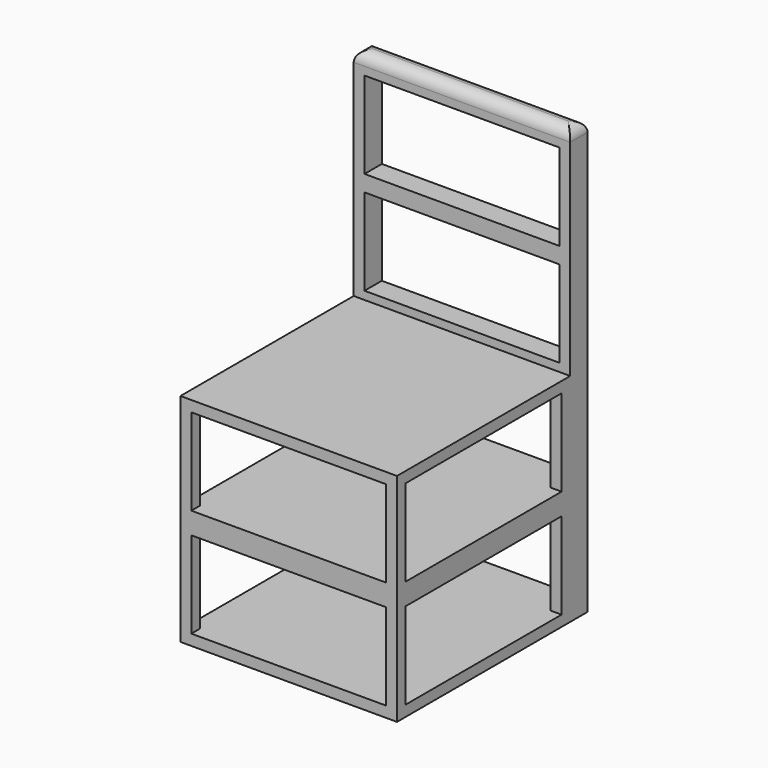
from build123d import *

# Parameters (mm, degrees)
F0_W     = 50
F0_H     = 5
F1_DEPTH = 100
F0_H_2   = 50
F2_DEPTH = 50
F3_W     = 22.5
F3_H     = 20
F4_DEPTH = 100
F5_W     = 22.5
F5_H     = 20
F6_DEPTH = 55
F7_R     = 2.49999
F8_W     = 45
F8_H     = 20
F9_DEPTH = 25


# Not quite as in the source:
# - a fillet or chamfer is up to 0.001 mm smaller than in the source, because OpenCascade refuses the exact size


with BuildPart() as f1:
    # F0 (on Top) → F1 (new body)
    with BuildSketch(Plane.XY):
        with Locations((0, 27.5)):
            Rectangle(F0_W, F0_H)
    extrude(amount=F1_DEPTH)

    # F0 (on Top) → F2 (join)
    with BuildSketch(Plane.XY):
        Rectangle(F0_W, F0_H_2)
    extrude(amount=F2_DEPTH)

    # F3 (on face) → F4 (cut)
    with BuildSketch(Plane.XZ.offset(25)):
        with Locations((-11.25, 37.5)):
            Rectangle(F3_W, F3_H)
        with Locations((11.25, 37.5)):
            Rectangle(F3_W, F3_H)
        with Locations((-11.25, 12.5)):
            Rectangle(F3_W, F3_H)
        with Locations((11.25, 12.5)):
            Rectangle(F3_W, F3_H)
    extrude(amount=-F4_DEPTH, mode=Mode.SUBTRACT)

    # F5 (on face) → F6 (cut)
    with BuildSketch(Plane(origin=(-25, 0, 0), x_dir=(0, -1, 0), z_dir=(-1, 0, 0))):
        with Locations((-11.25, 37.5)):
            Rectangle(F5_W, F5_H)
        with Locations((11.25, 37.5)):
            Rectangle(F5_W, F5_H)
        with Locations((11.25, 12.5)):
            Rectangle(F5_W, F5_H)
        with Locations((-11.25, 12.5)):
            Rectangle(F5_W, F5_H)
    extrude(amount=-F6_DEPTH, mode=Mode.SUBTRACT)

    # F7 (radius 2.5 in the source; OpenCascade refuses exactly that, so slightly less here)
    f7_edges = [f1.edges().sort_by_distance(p)[0] for p in [
        (0, 25, 100),
        (25, 27.5, 100),
        (0, 30, 100),
        (-25, 27.5, 100),
    ]]
    fillet(f7_edges, radius=F7_R)

    # F8 (on face) → F9 (cut)
    with BuildSketch(Plane.XZ.offset(-25)):
        with Locations((0, 85.625)):
            Rectangle(F8_W, F8_H)
        with Locations((0, 61.875)):
            Rectangle(F8_W, F8_H)
    extrude(amount=-F9_DEPTH, mode=Mode.SUBTRACT)


solid = f1.part
